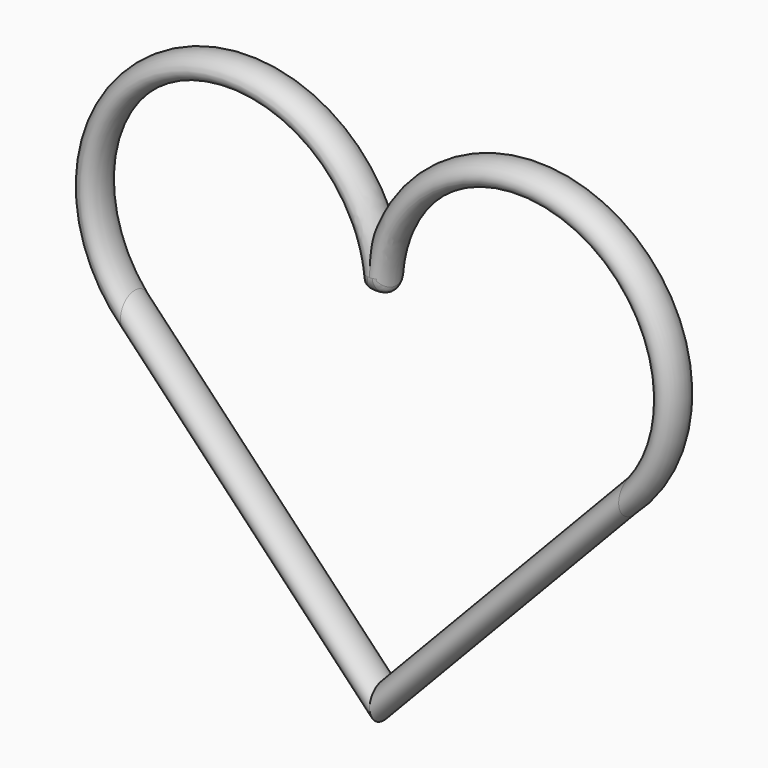
from build123d import *

# Parameters (mm, degrees)
F1_R          = 0.635
F5_ANGLE_BACK = 90
F5_ANGLE      = 180
F6_R          = 0.254


with BuildPart() as f2:
    # F2: sweep along a path in F0
    with BuildLine(Plane.XZ) as f2_path:
        Line((0, -9.1965517241), (-8.7586206897, 0))
        ThreePointArc((-8.7586206897, 0), (-6.9666646359, 8.2201098656), (0, 3.5034482759))
    # F1 (on Right) → F2 (sweep)
    with BuildSketch(Plane.YZ):
        with Locations((0, -9.1965517241)):
            Circle(F1_R)
    sweep(path=f2_path.line)

    # F3: sweep along a path in F0
    with BuildLine(Plane.XZ) as f3_path:
        Line((0, -9.1965517241), (8.7586206897, 0))
        ThreePointArc((8.7586206897, 0), (6.9666646359, 8.2201098656), (0, 3.5034482759))
    # F1 (on Right) → F3 (sweep)
    with BuildSketch(Plane.YZ):
        with Locations((0, -9.1965517241)):
            Circle(F1_R)
    sweep(path=f3_path.line)

    # F4 (on Front) → F5 (revolve, cut)
    with BuildSketch(Plane.XZ, mode=Mode.PRIVATE) as f5_sk:
        with BuildLine():
            Line((1.3799275509, 4.132134429), (0.939278438, 4.132134429))
            ThreePointArc((0.939278438, 4.132134429), (0, 3.5034482759), (-0.939278438, 4.132134429))
            Line((-0.939278438, 4.132134429), (-1.2599644945, 4.132134429))
            Line((-1.2599644945, 4.132134429), (-1.2599644945, 2.9368885409))
            Line((-1.2599644945, 2.9368885409), (1.3799275509, 2.9368885409))
            Line((1.3799275509, 2.9368885409), (1.3799275509, 4.132134429))
        make_face()
    revolve(f5_sk.sketch.rotate(Axis((0, 0, 4.132134429), (-1, 0, 0)), -F5_ANGLE_BACK), axis=Axis((0, 0, 4.132134429), (-1, 0, 0)), revolution_arc=F5_ANGLE, mode=Mode.SUBTRACT)

    # F6
    f6_edges = [f2.edges().sort_by_distance(p)[0] for p in [
        (-0.416063, 0, 3.592546),
        (0.416063, 0, 3.592546),
    ]]
    fillet(f6_edges, radius=F6_R)


solid = f2.part
